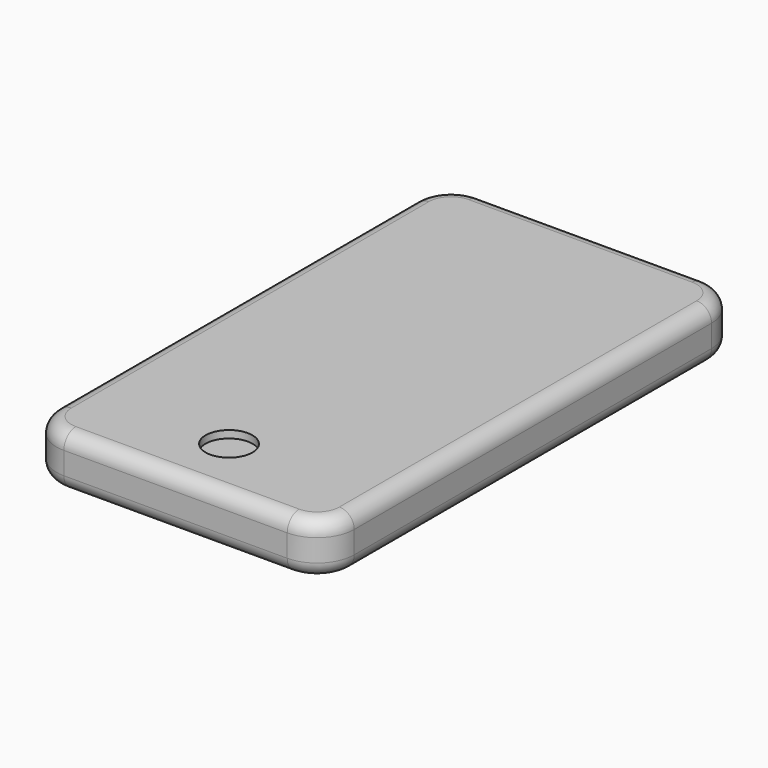
from build123d import *

# Parameters (mm, degrees)
F0_W         = 40
F0_H         = 70
F1_DEPTH     = 7
F2_R         = 5
F3_R         = 2.0663885281
F4_DEPTH     = 5
F5_T1_DEPTH  = 60
F5_T3_DEPTH  = 30
F5_T6_ANGLE  = 90
F5_T8_ANGLE  = 90
F5_T10_ANGLE = 90
F5_T12_ANGLE = 90
F5_T14_ANGLE = 90
F5_T16_ANGLE = 90
F5_T18_ANGLE = 90
F5_T20_ANGLE = 90
F6_R         = 3.1424887648
F7_DEPTH     = 1


# Not quite as in the source:
# - a fillet or chamfer that OpenCascade refuses, or shapes differently, is made with other operations: its cross-section is extruded or revolved along the edge and cut away or added


with BuildPart() as f1:
    # F0 (on Top) → F1 (new body)
    with BuildSketch(Plane.XY):
        with Locations((20, 35)):
            Rectangle(F0_W, F0_H)
    extrude(amount=F1_DEPTH)

    # F2
    f2_edges = [f1.edges().sort_by_distance(p)[0] for p in [
        (40, 0, 3.5),
        (40, 70, 3.5),
        (0, 0, 3.5),
        (0, 70, 3.5),
    ]]
    fillet(f2_edges, radius=F2_R)

    # F3 (on face) → F4 (cut)
    with BuildSketch(Plane(origin=(0, 70, 0), x_dir=(-1, 0, 0), z_dir=(0, 1, 0))):
        with Locations((-29.0856193751, 3.5)):
            Circle(F3_R)
    extrude(amount=-F4_DEPTH, mode=Mode.SUBTRACT)

    # F5: fillet of radius 2 on 16 edges, made by hand

    # F5_s2 → F5_t1 (cut)
    with BuildSketch(Plane.XZ.offset(-65)):
        with BuildLine():
            ThreePointArc((2, 7), (0.5857864376, 6.4142135624), (0, 5))
            Line((0, 5), (0, 7))
            Line((0, 7), (2, 7))
        make_face()
        with BuildLine():
            ThreePointArc((2, 0), (0.5857864376, 0.5857864376), (0, 2))
            Line((0, 2), (0, 0))
            Line((0, 0), (2, 0))
        make_face()
        with BuildLine():
            ThreePointArc((38, 0), (39.4142135624, 0.5857864376), (40, 2))
            Line((40, 2), (40, 0))
            Line((40, 0), (38, 0))
        make_face()
        with BuildLine():
            ThreePointArc((38, 7), (39.4142135624, 6.4142135624), (40, 5))
            Line((40, 5), (40, 7))
            Line((40, 7), (38, 7))
        make_face()
    extrude(amount=F5_T1_DEPTH, mode=Mode.SUBTRACT)

    # F5_s4 → F5_t3 (cut)
    with BuildSketch(Plane.YZ.offset(5)):
        with BuildLine():
            ThreePointArc((70, 2), (69.4142135624, 0.5857864376), (68, 0))
            Line((68, 0), (70, 0))
            Line((70, 0), (70, 2))
        make_face()
        with BuildLine():
            ThreePointArc((70, 5), (69.4142135624, 6.4142135624), (68, 7))
            Line((68, 7), (70, 7))
            Line((70, 7), (70, 5))
        make_face()
        with BuildLine():
            ThreePointArc((2, 0), (0.5857864376, 0.5857864376), (0, 2))
            Line((0, 2), (0, 0))
            Line((0, 0), (2, 0))
        make_face()
        with BuildLine():
            ThreePointArc((2, 7), (0.5857864376, 6.4142135624), (0, 5))
            Line((0, 5), (0, 7))
            Line((0, 7), (2, 7))
        make_face()
    extrude(amount=F5_T3_DEPTH, mode=Mode.SUBTRACT)

    # F5_s5 → F5_t6 (revolve, cut)
    with BuildSketch(Plane.YZ.offset(35)):
        with BuildLine():
            ThreePointArc((68, 0), (69.4142135624, 0.5857864376), (70, 2))
            Line((70, 2), (70, 0))
            Line((70, 0), (68, 0))
        make_face()
    revolve(axis=Axis((35, 65, 0), (0, 0, -1)), revolution_arc=F5_T6_ANGLE, mode=Mode.SUBTRACT)

    # F5_s7 → F5_t8 (revolve, cut)
    with BuildSketch(Plane.YZ.offset(5)):
        with BuildLine():
            ThreePointArc((68, 0), (69.4142135624, 0.5857864376), (70, 2))
            Line((70, 2), (70, 0))
            Line((70, 0), (68, 0))
        make_face()
    revolve(axis=Axis((5, 65, 0), (0, 0, 1)), revolution_arc=F5_T8_ANGLE, mode=Mode.SUBTRACT)

    # F5_s9 → F5_t10 (revolve, cut)
    with BuildSketch(Plane.YZ.offset(35)):
        with BuildLine():
            ThreePointArc((2, 0), (0.5857864376, 0.5857864376), (0, 2))
            Line((0, 2), (0, 0))
            Line((0, 0), (2, 0))
        make_face()
    revolve(axis=Axis((35, 5, 0), (0, 0, 1)), revolution_arc=F5_T10_ANGLE, mode=Mode.SUBTRACT)

    # F5_s11 → F5_t12 (revolve, cut)
    with BuildSketch(Plane.XZ.offset(-5)):
        with BuildLine():
            ThreePointArc((2, 0), (0.5857864376, 0.5857864376), (0, 2))
            Line((0, 2), (0, 0))
            Line((0, 0), (2, 0))
        make_face()
    revolve(axis=Axis((5, 5, 0), (0, 0, 1)), revolution_arc=F5_T12_ANGLE, mode=Mode.SUBTRACT)

    # F5_s13 → F5_t14 (revolve, cut)
    with BuildSketch(Plane.YZ.offset(35)):
        with BuildLine():
            ThreePointArc((70, 5), (69.4142135624, 6.4142135624), (68, 7))
            Line((68, 7), (70, 7))
            Line((70, 7), (70, 5))
        make_face()
    revolve(axis=Axis((35, 65, 7), (0, 0, -1)), revolution_arc=F5_T14_ANGLE, mode=Mode.SUBTRACT)

    # F5_s15 → F5_t16 (revolve, cut)
    with BuildSketch(Plane.YZ.offset(5)):
        with BuildLine():
            ThreePointArc((70, 5), (69.4142135624, 6.4142135624), (68, 7))
            Line((68, 7), (70, 7))
            Line((70, 7), (70, 5))
        make_face()
    revolve(axis=Axis((5, 65, 7), (0, 0, 1)), revolution_arc=F5_T16_ANGLE, mode=Mode.SUBTRACT)

    # F5_s17 → F5_t18 (revolve, cut)
    with BuildSketch(Plane.YZ.offset(35)):
        with BuildLine():
            ThreePointArc((2, 7), (0.5857864376, 6.4142135624), (0, 5))
            Line((0, 5), (0, 7))
            Line((0, 7), (2, 7))
        make_face()
    revolve(axis=Axis((35, 5, 7), (0, 0, 1)), revolution_arc=F5_T18_ANGLE, mode=Mode.SUBTRACT)

    # F5_s19 → F5_t20 (revolve, cut)
    with BuildSketch(Plane.XZ.offset(-5)):
        with BuildLine():
            ThreePointArc((2, 7), (0.5857864376, 6.4142135624), (0, 5))
            Line((0, 5), (0, 7))
            Line((0, 7), (2, 7))
        make_face()
    revolve(axis=Axis((5, 5, 7), (0, 0, 1)), revolution_arc=F5_T20_ANGLE, mode=Mode.SUBTRACT)

    # F6 (on face) → F7 (cut)
    with BuildSketch(Plane.XY.offset(7)):
        with Locations((20, 8.9777829126)):
            Circle(F6_R)
    extrude(amount=-F7_DEPTH, mode=Mode.SUBTRACT)


solid = f1.part
